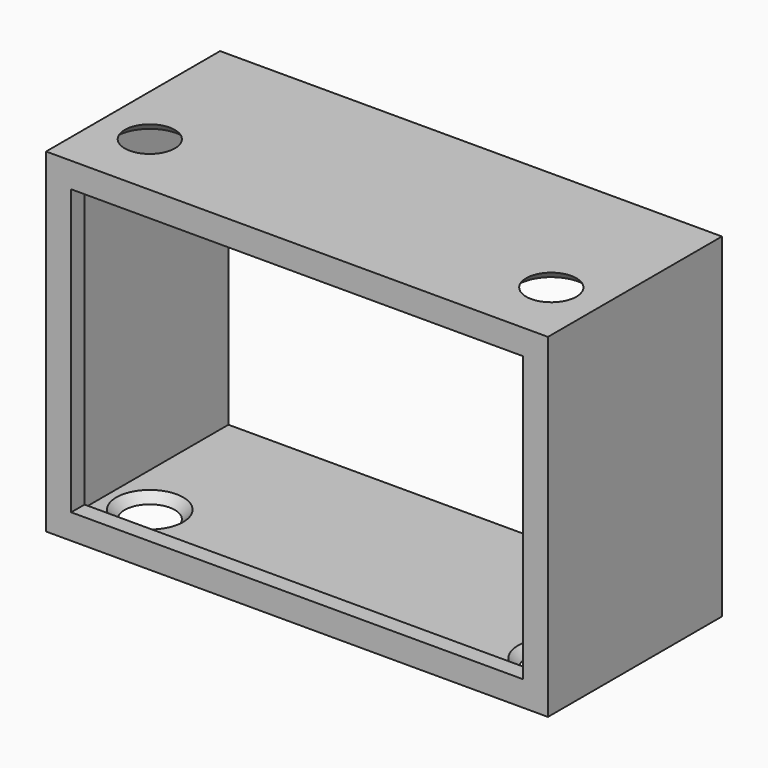
from build123d import *

# Parameters (mm, degrees)
F0_W     = 30
F0_H     = 12
F0_R     = 1.5
F1_DEPTH = 20
F2_W     = 29
F2_H     = 19
F2_W_2   = 27
F2_H_2   = 17
F3_DEPTH = 12
F2_W_3   = 30
F2_H_3   = 20
F4_DEPTH = 1
F5_SIZE2 = 0.49999
F5_SIZE  = 0.49999


# Not quite as in the source:
# - a fillet or chamfer is up to 0.001 mm smaller than in the source, because OpenCascade refuses the exact size


with BuildPart() as f1:
    # F0 (on Top) → F1 (new body)
    with BuildSketch(Plane.XY):
        with Locations((0, 6)):
            Rectangle(F0_W, F0_H)
        with Locations((-12, 3)):
            Circle(F0_R, mode=Mode.SUBTRACT)
        with Locations((12, 3)):
            Circle(F0_R, mode=Mode.SUBTRACT)
    extrude(amount=F1_DEPTH)

    # F2 (on Front) → F3 (cut)
    with BuildSketch(Plane.XZ):
        with Locations((0, 10)):
            Rectangle(F2_W, F2_H)
        with Locations((0, 10)):
            Rectangle(F2_W_2, F2_H_2, mode=Mode.SUBTRACT)
        with Locations((0, 10)):
            Rectangle(F2_W_2, F2_H_2)
    extrude(amount=-F3_DEPTH, mode=Mode.SUBTRACT)

    # F2 (on Front) → F4 (join)
    with BuildSketch(Plane.XZ):
        with Locations((0, 10)):
            Rectangle(F2_W_3, F2_H_3)
        with Locations((0, 10)):
            Rectangle(F2_W, F2_H, mode=Mode.SUBTRACT)
        with Locations((0, 10)):
            Rectangle(F2_W, F2_H)
        with Locations((0, 10)):
            Rectangle(F2_W_2, F2_H_2, mode=Mode.SUBTRACT)
    extrude(amount=F4_DEPTH)

    # F5 (size 0.5 and 0.5 in the source; OpenCascade refuses exactly that, so slightly less here)
    f5_edges = [f1.edges().sort_by_distance(p)[0] for p in [
        (-13.5, 3, 0.5),
        (10.5, 3, 0.5),
        (10.5, 3, 19.5),
        (-13.5, 3, 19.5),
    ]]
    chamfer(f5_edges, length=F5_SIZE, length2=F5_SIZE2)


solid = f1.part
